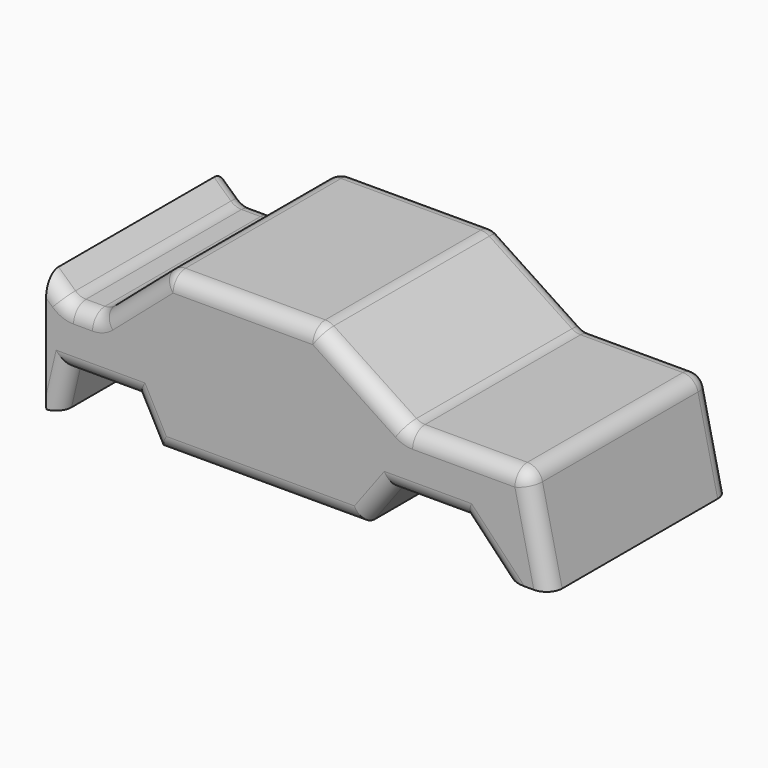
from build123d import *

# Parameters (mm, degrees)
F1_DEPTH = 73.66
F2_R     = 5.08


with BuildPart() as f1:
    # F0 (on Front) → F1 (new body)
    with BuildSketch(Plane.XZ):
        Polygon((-94.9451997876, 22.5552003831), (-94.9451997876, -16.4592005312), (-90.67799896, -16.4592005312), (-87.6299962401, -3.3528001513), (-65.6844004989, -3.3528001513), (-58.6740002036, -16.4592005312), (8.3820000291, -16.4592005312), (18.1356016546, -3.3528001513), (41.9100001454, -3.3528001513), (54.406799376, -16.4592005312), (69.6468055248, -16.4592005312), (62.3316019773, 16.1543991417), (23.3171992004, 16.1543991417), (-6.2483996153, 35.6616005301), (-55.3212016821, 35.6616005301), (-77.8764039278, 16.1543991417), (-87.9347994924, 16.1543991417), align=None)
    extrude(amount=F1_DEPTH)

    # F2
    f2_edges = [f1.edges().sort_by_distance(p)[0] for p in [
        (65.989204, 0, -0.152401),
        (62.331602, -36.83, 16.154399),
        (65.989204, -73.66, -0.152401),
        (42.824401, 0, 16.154399),
        (8.5344, 0, 25.908),
        (-6.2484, -36.83, 35.661601),
        (8.5344, -73.66, 25.908),
        (42.824401, -73.66, 16.154399),
        (23.317199, -36.83, 16.154399),
        (-30.784801, 0, 35.661601),
        (-55.321202, -36.83, 35.661601),
        (-30.784801, -73.66, 35.661601),
        (-66.598803, -73.66, 25.908),
        (-77.876404, -36.83, 16.154399),
        (-66.598803, 0, 25.908),
        (-82.905602, 0, 16.154399),
        (-87.934799, -36.83, 16.154399),
        (-89.153998, -73.66, -9.906),
        (-76.657198, -73.66, -3.3528),
        (-62.1792, -73.66, -9.906),
        (-25.146, -73.66, -16.459201),
        (13.258801, -73.66, -9.906),
        (30.022801, -73.66, -3.3528),
        (48.1584, -73.66, -9.906),
        (-82.905602, -73.66, 16.154399),
        (-91.44, 0, 19.3548),
        (-91.44, -73.66, 19.3548),
    ]]
    fillet(f2_edges, radius=F2_R)


solid = f1.part
